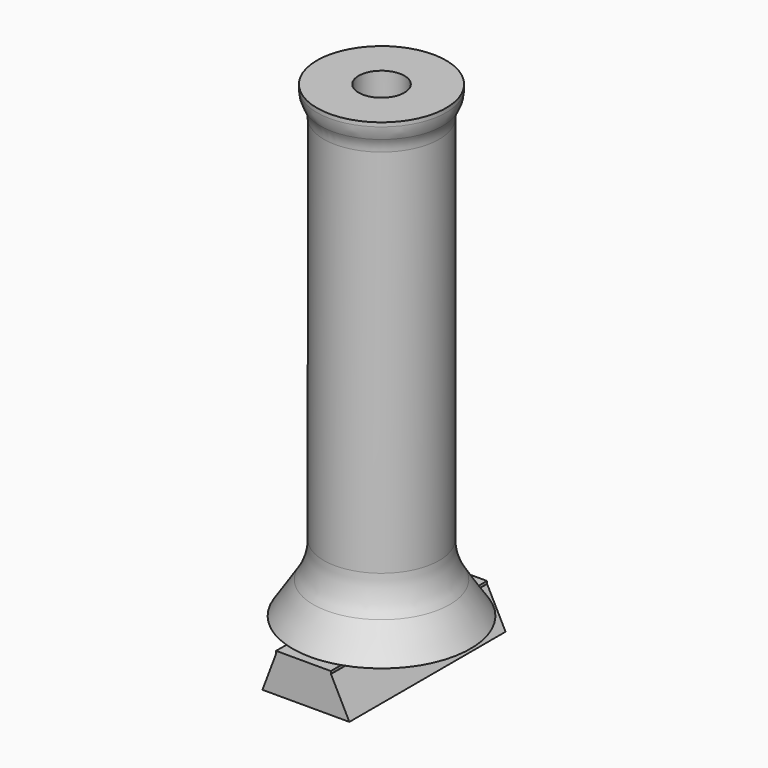
from build123d import *

# Parameters (mm, degrees)
F1_DEPTH    = 7.5
F3_R        = 5
F4_S5_R     = 4.9585432895
F4_T6_DEPTH = 9
F5_R        = 2


# Not quite as in the source:
# - a fillet or chamfer that OpenCascade refuses, or shapes differently, is made with other operations: its cross-section is extruded or revolved along the edge and cut away or added
# - a feature names something its author has since deleted; it is built from what else it names


with BuildPart() as f1:
    # F0 (on Front) → F1 (new body, symmetric)
    with BuildSketch(Plane.XZ):
        Polygon((-2.3518713359, 1.3106813192), (-2.3518713359, 1.1106813192), (1.854373375, 1.1106813192), (1.854373375, 1.3106813192), (-0.2487489805, 1.3106813192), align=None)
        Polygon((-3.3989118356, -1.6660219789), (3.2814688813, -1.6660219789), (1.8650586641, 1.1106813192), (1.854373375, 1.1106813192), (-2.3518713359, 1.1106813192), align=None)
    extrude(amount=F1_DEPTH, both=True)

    # F0 (on Front) → F2 (revolve)
    with BuildSketch(Plane.XZ):
        Polygon((-7.0862104185, 1.3106813192), (-2.3518713359, 1.3106813192), (-0.2487489805, 1.3106813192), (-0.2487489805, 3.5361030605), (-2.0069789607, 3.5361030605), (-2.0069789607, 37.2762935372), (-5.2072922699, 37.2762935372), (-5.2072922699, 36.3391824067), (-4.6829497442, 35.7728934956), (-4.6829497442, 5.0174454227), align=None)
    revolve(axis=Axis((-0.2487489805, 0, -2.0752633687), (0, 0, -1)))

    # F3
    f3_edges = [f1.edges().sort_by_distance(p)[0] for p in [
        (4.185452, 0, 5.017445),
    ]]
    fillet(f3_edges, radius=F3_R)

    # F4: fillet of radius 2 on 1 edges, made by hand


with BuildPart() as f4_tool2:
    # F4_s3 → F4_t4 (revolve)
    with BuildSketch(Plane.XZ):
        with BuildLine():
            ThreePointArc((-4.6829497442, 34.9891533442), (-4.8208218936, 35.718865526), (-5.2154296124, 36.3479707207))
            Line((-5.2154296124, 36.3479707207), (-4.6829497442, 35.7728934956))
            Line((-4.6829497442, 35.7728934956), (-4.6829497442, 34.9891533442))
        make_face()
    revolve(axis=Axis((-0.2487489805, 0, 35.7728934956), (0, 0, -1)))

    # F4_s5 → F4_t6 (intersect, symmetric)
    with BuildSketch(Plane.XY.offset(35.7)):
        with Locations((-0.2487489805, 0)):
            Circle(F4_S5_R)
    extrude(amount=F4_T6_DEPTH, both=True, mode=Mode.INTERSECT)


with BuildPart() as f1_1:
    add(f1.part)

    # F4_t1: union F4_tool2
    add(f4_tool2.part)

    # F5
    f5_edges = [f1_1.edges().sort_by_distance(p)[0] for p in [
        (-0.248749, 4.958543, 36.339129),
        (-0.248749, -4.958543, 36.339129),
    ]]
    fillet(f5_edges, radius=F5_R)


solid = f1_1.part
